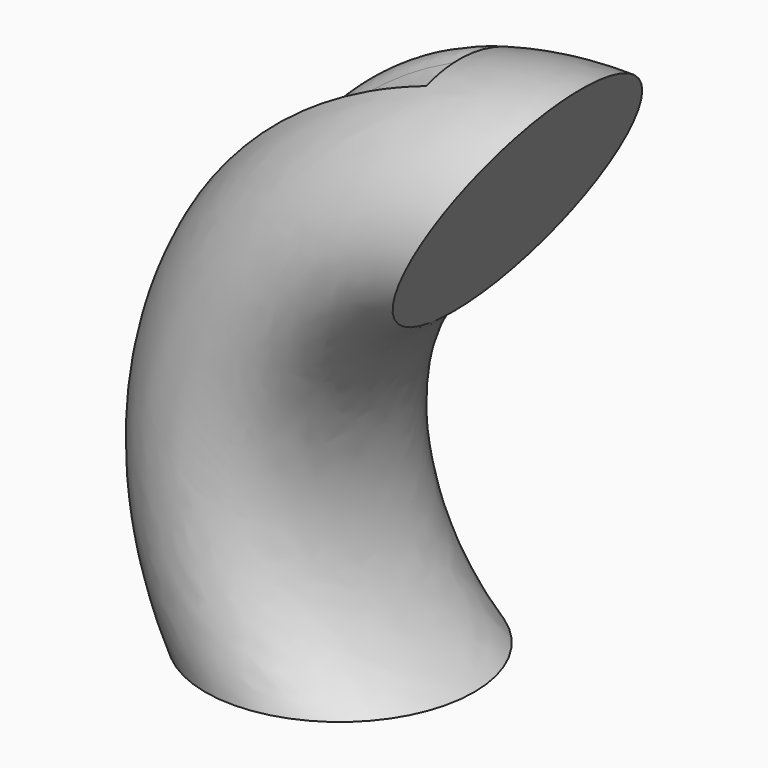
from build123d import *

# Parameters (mm, degrees)
F0_R = 17.0508344958
F3_R = 6.5798562112
F6_R = 2.54


with BuildPart() as f2:
    # F2: sweep along a path in F1
    with BuildLine(Plane.XZ) as f2_path:
        ThreePointArc((22.5486494601, 56.7756593227), (-4.8260451433, 34.7821472401), (0, 0))
    # F0 (on Top) → F2 (sweep)
    with BuildSketch(Plane.XY):
        Circle(F0_R)
    sweep(path=f2_path.line)

    # F5: sweep along a path in F4
    with BuildLine(Plane.XZ) as f5_path:
        ThreePointArc((14.7513579577, 73.1248388765), (-16.9846248554, 43.3251523108), (-21.2419833988, 0))
    # F3 (on Top) → F5 (sweep, cut)
    with BuildSketch(Plane.XY):
        with Locations((-21.2419833988, 0)):
            Circle(F3_R)
    sweep(path=f5_path.line, mode=Mode.SUBTRACT)

    # F6
    f6_edges = [f2.edges().sort_by_distance(p)[0] for p in [
        (-16.429502, 6.477089, 41.900907),
    ]]
    fillet(f6_edges, radius=F6_R)


solid = f2.part
